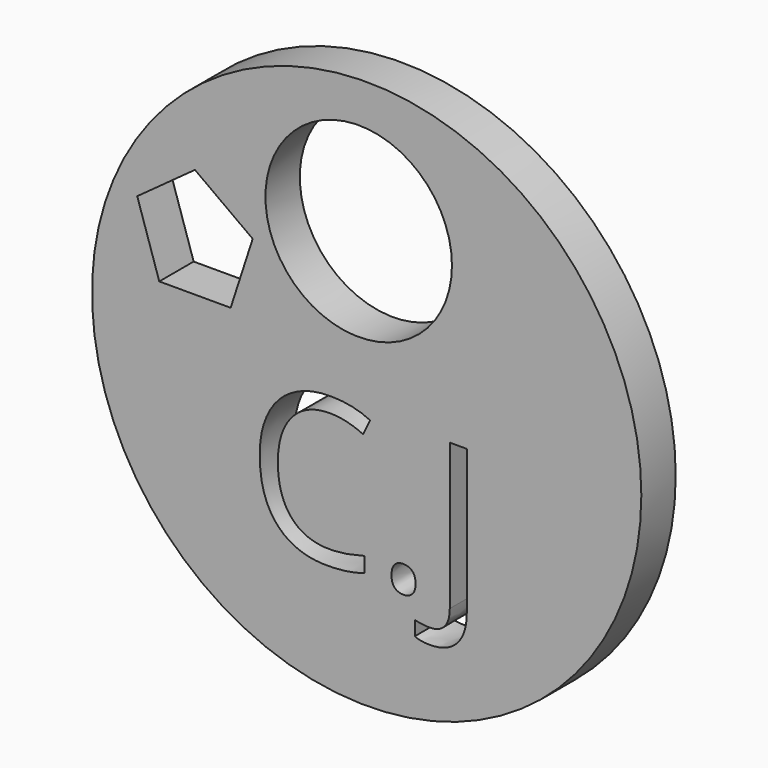
from build123d import *

# Parameters (mm, degrees)
F0_R         = 13.737496768
F1_DEPTH     = 2.15
F2_R         = 4.6644030248
F3_DEPTH     = 2.15
F4_TEXT_SIZE = 10.236136667
F5_DEPTH     = 2.15
F7_DEPTH     = 2.15


# Not quite as in the source:
# - Text() gives the source's letters only with a copy of the font that has no kerning and outlines rounded to 1/6400 em; it was checked with that copy


with BuildPart() as f1:
    # F0 (on Front) → F1 (new body)
    with BuildSketch(Plane.XZ):
        with Locations((-26.6237780452, 21.0771579295)):
            Circle(F0_R)
    extrude(amount=F1_DEPTH)

    # F2 (on Front) → F3 (cut, through all)
    with BuildSketch(Plane.XZ):
        with Locations((-27.0233973861, 28.1152520329)):
            Circle(F2_R)
    extrude(amount=F3_DEPTH, mode=Mode.SUBTRACT)

    # F4 (on Front) → F5 (cut, through all)
    with BuildSketch(Plane.XZ):
        with Locations((-32.5992014259, 12.9778189585)):
            Text('C.J', F4_TEXT_SIZE, font='Open Sans', text_align=(TextAlign.LEFT, TextAlign.BOTTOM))
    extrude(amount=F5_DEPTH, mode=Mode.SUBTRACT)

    # F6 (on Front) → F7 (cut, through all)
    with BuildSketch(Plane.XZ):
        Polygon((-36.9971828375, 22.6559787989), (-33.4274260487, 22.6559787989), (-32.3243105352, 26.0510192544), (-35.2123044431, 28.1492696492), (-38.100298351, 26.0510192544), align=None)
    extrude(amount=F7_DEPTH, mode=Mode.SUBTRACT)


solid = f1.part
